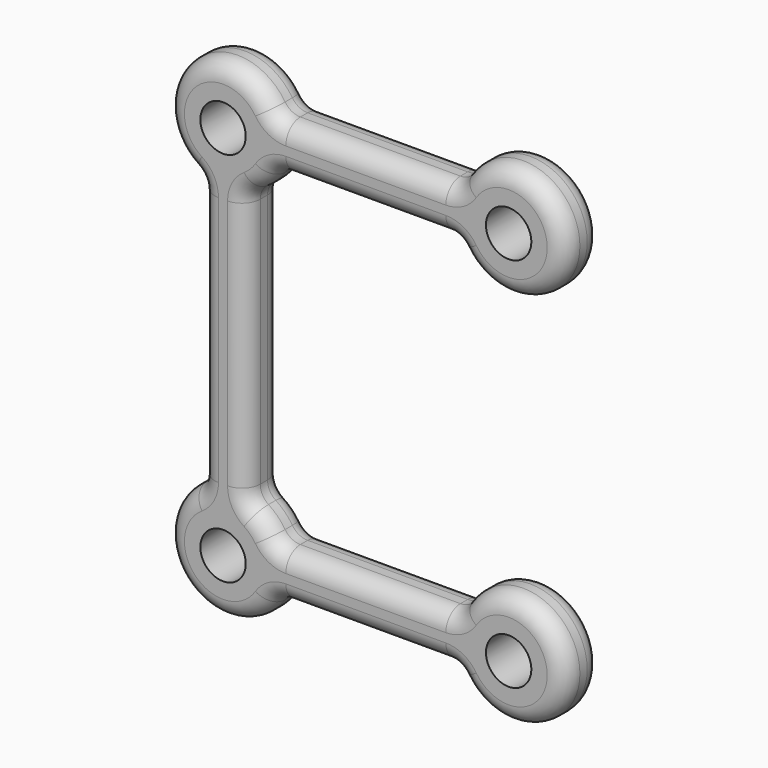
from build123d import *

# Parameters (mm, degrees)
F1_DEPTH = 6.35
F2_DEPTH = 6.35
F3_R     = 5.08
F4_R     = 6.35
F5_DEPTH = 12.701


with BuildPart() as f1:
    # F0 (on Front) → F1 (new body, symmetric)
    with BuildSketch(Plane.XZ):
        with BuildLine():
            ThreePointArc((-21.7996303504, 64.6400047008), (-20.8091704641, 67.7465891072), (-20.4743081819, 70.9900047008))
            ThreePointArc((-20.4743081819, 70.9900047008), (-20.8091704641, 74.2334202943), (-21.7996303504, 77.3400047008))
            ThreePointArc((-21.7996303504, 77.3400047008), (-47.5746283332, 82.2153248521), (-42.6993081819, 56.4403268693))
            ThreePointArc((-42.6993081819, 56.4403268693), (-36.3493081819, 55.1150047008), (-29.9993081819, 56.4403268693))
            ThreePointArc((-29.9993081819, 56.4403268693), (-25.1239880306, 59.7646845494), (-21.7996303504, 64.6400047008))
        make_face()
        with BuildLine():
            ThreePointArc((-21.7996303504, 77.3400047008), (-20.8091704641, 74.2334202943), (-20.4743081819, 70.9900047008))
            ThreePointArc((-20.4743081819, 70.9900047008), (-20.8091704641, 67.7465891072), (-21.7996303504, 64.6400047008))
            Line((-21.7996303504, 64.6400047008), (29.0003696496, 64.6400047008))
            ThreePointArc((29.0003696496, 64.6400047008), (27.6750474811, 70.9900047008), (29.0003696496, 77.3400047008))
            Line((29.0003696496, 77.3400047008), (-21.7996303504, 77.3400047008))
        make_face()
        with BuildLine():
            ThreePointArc((29.0003696496, -27.9593509622), (27.6750474811, -34.3093509622), (29.0003696496, -40.6593509622))
            ThreePointArc((29.0003696496, -40.6593509622), (46.7934630746, -49.84948868), (59.4250474811, -34.3093509622))
            ThreePointArc((59.4250474811, -34.3093509622), (46.7934630746, -18.7692132444), (29.0003696496, -27.9593509622))
        make_face()
        with BuildLine():
            ThreePointArc((-20.4743081819, -34.3093509622), (-20.8091704641, -37.5527665558), (-21.7996303504, -40.6593509622))
            Line((-21.7996303504, -40.6593509622), (29.0003696496, -40.6593509622))
            ThreePointArc((29.0003696496, -40.6593509622), (27.6750474811, -34.3093509622), (29.0003696496, -27.9593509622))
            Line((29.0003696496, -27.9593509622), (-21.7996303504, -27.9593509622))
            ThreePointArc((-21.7996303504, -27.9593509622), (-20.8091704641, -31.0659353686), (-20.4743081819, -34.3093509622))
        make_face()
        with BuildLine():
            ThreePointArc((-29.9993081819, -19.7596731307), (-36.3493081819, -18.4343509622), (-42.6993081819, -19.7596731307))
            ThreePointArc((-42.6993081819, -19.7596731307), (-47.5746283332, -45.5346711135), (-21.7996303504, -40.6593509622))
            ThreePointArc((-21.7996303504, -40.6593509622), (-20.8091704641, -37.5527665558), (-20.4743081819, -34.3093509622))
            ThreePointArc((-20.4743081819, -34.3093509622), (-20.8091704641, -31.0659353686), (-21.7996303504, -27.9593509622))
            ThreePointArc((-21.7996303504, -27.9593509622), (-25.1239880306, -23.0840308109), (-29.9993081819, -19.7596731307))
        make_face()
        with BuildLine():
            ThreePointArc((-29.9993081819, 56.4403268693), (-36.3493081819, 55.1150047008), (-42.6993081819, 56.4403268693))
            Line((-42.6993081819, 56.4403268693), (-42.6993081819, -19.7596731307))
            ThreePointArc((-42.6993081819, -19.7596731307), (-36.3493081819, -18.4343509622), (-29.9993081819, -19.7596731307))
            Line((-29.9993081819, -19.7596731307), (-29.9993081819, 56.4403268693))
        make_face()
    extrude(amount=F1_DEPTH, both=True)

    # F0 (on Front) → F2 (join, symmetric)
    with BuildSketch(Plane.XZ):
        with BuildLine():
            ThreePointArc((59.4250474811, 70.9900047008), (46.7934630746, 86.5301424186), (29.0003696496, 77.3400047008))
            ThreePointArc((29.0003696496, 77.3400047008), (27.6750474811, 70.9900047008), (29.0003696496, 64.6400047008))
            ThreePointArc((29.0003696496, 64.6400047008), (46.7934630746, 55.449866983), (59.4250474811, 70.9900047008))
        make_face()
    extrude(amount=F2_DEPTH, both=True)

    # F3
    f3_edges = [f1.edges().sort_by_distance(p)[0] for p in [
        (29.00037, 0, 77.340005),
        (3.60037, 6.35, 77.340005),
        (-21.79963, 0, 77.340005),
        (3.60037, -6.35, 77.340005),
        (-47.574628, 6.35, 82.215325),
        (-42.699308, 0, 56.440327),
        (-47.574628, -6.35, 82.215325),
        (29.00037, 0, 64.640005),
        (59.425047, 6.35, 70.990005),
        (59.425047, -6.35, 70.990005),
        (-25.123988, -6.35, 59.764685),
        (-25.123988, 6.35, 59.764685),
        (-21.79963, 0, 64.640005),
        (-29.999308, 0, 56.440327),
        (3.60037, -6.35, 64.640005),
        (-42.699308, -6.35, 18.340327),
        (-47.574628, -6.35, -45.534671),
        (3.60037, -6.35, -40.659351),
        (59.425047, -6.35, -34.309351),
        (3.60037, -6.35, -27.959351),
        (-25.123988, -6.35, -23.084031),
        (-29.999308, -6.35, 18.340327),
        (3.60037, 6.35, 64.640005),
        (-42.699308, 6.35, 18.340327),
        (-47.574628, 6.35, -45.534671),
        (3.60037, 6.35, -40.659351),
        (59.425047, 6.35, -34.309351),
        (3.60037, 6.35, -27.959351),
        (-25.123988, 6.35, -23.084031),
        (-29.999308, 6.35, 18.340327),
        (29.00037, 0, -40.659351),
        (29.00037, 0, -27.959351),
        (-21.79963, 0, -27.959351),
        (-29.999308, 0, -19.759673),
        (-42.699308, 0, -19.759673),
        (-21.79963, 0, -40.659351),
    ]]
    fillet(f3_edges, radius=F3_R)

    # F4 (on face) → F5 (cut, through all)
    with BuildSketch(Plane.XZ.offset(6.35)):
        with Locations((-36.3493081819, 70.9900047008)):
            Circle(F4_R)
        with Locations((43.5500474811, 70.9900047008)):
            Circle(F4_R)
        with Locations((-36.3493081819, -34.3093509622)):
            Circle(F4_R)
        with Locations((43.5500474811, -34.3093509622)):
            Circle(F4_R)
    extrude(amount=-F5_DEPTH, mode=Mode.SUBTRACT)


with BuildPart() as f1_1:
    # F6: moved
    add(f1.part.moved(Location((0, -25.4, 0))))


solid = f1_1.part
